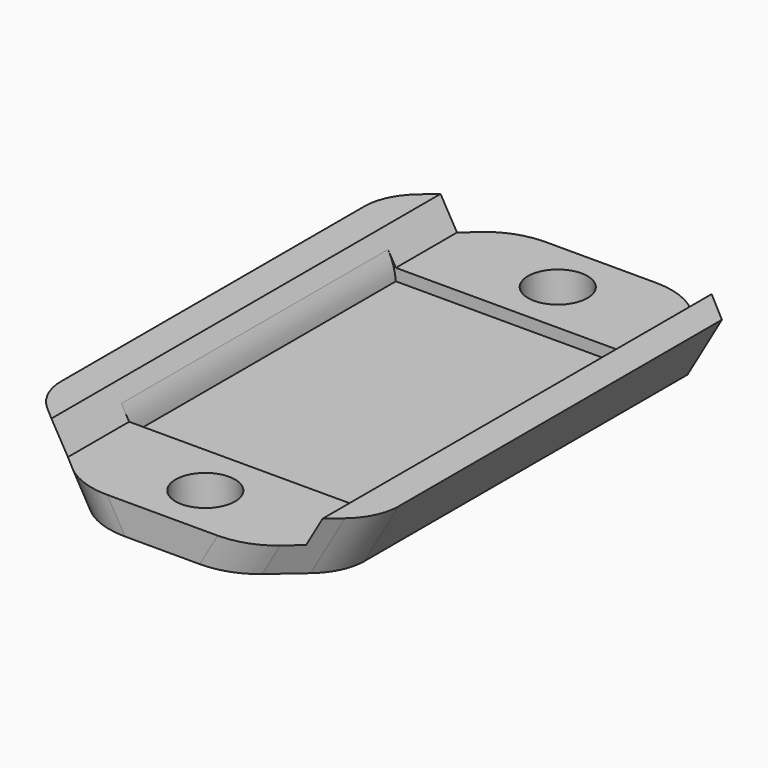
from build123d import *

# Parameters (mm, degrees)
F1_DEPTH    = 23
F2_W        = 20
F2_H        = 28
F3_DEPTH    = 1
F4_D        = 5
F5_SIZE     = 5
F6_T1_DEPTH = 28
F6_T3_DEPTH = 13.3575604591
F6_T5_DEPTH = 13.3575604591
F6_T7_DEPTH = 16.1288417512
F6_T9_DEPTH = 16.1288417512


# Not quite as in the source:
# - a fillet or chamfer that OpenCascade refuses, or shapes differently, is made with other operations: its cross-section is extruded or revolved along the edge and cut away or added


with BuildPart() as f1:
    # F0 (on Front) → F1 (new body, symmetric)
    with BuildSketch(Plane.XZ):
        Polygon((-11.2988893001, 0), (0, 0), (11.2988893001, 0), (14.1856406461, 5), (11.3856406461, 5), (10, 2.6), (0, 2.6), (-10, 2.6), (-11.3856406461, 5), (-14.1856406461, 5), align=None)
    extrude(amount=F1_DEPTH, both=True)

    # F2 (on face) → F3 (cut)
    with BuildSketch(Plane.XY.offset(2.6)):
        Rectangle(F2_W, F2_H)
    extrude(amount=-F3_DEPTH, mode=Mode.SUBTRACT)

    # F4 (through all)
    with Locations(Plane.XY.offset(2.6)):
        with Locations((0, -18.5), (0, 18.5)):
            Hole(F4_D / 2)

    # F5
    f5_edges = [f1.edges().sort_by_distance(p)[0] for p in [
        (-12.742265, -23, 2.5),
        (12.742265, -23, 2.5),
        (-12.742265, 23, 2.5),
        (12.742265, 23, 2.5),
    ]]
    chamfer(f5_edges, length=F5_SIZE)

    # F6: fillet of radius 5 on 9 edges, made by hand

    # F6_s2 → F6_t1 (cut)
    with BuildSketch(Plane.XZ.offset(-14)):
        with BuildLine():
            ThreePointArc((-10.656712034, 3.7374586088), (-10.2073363045, 2.7059113585), (-10, 1.6))
            Line((-10, 1.6), (-10, 2.6))
            Line((-10, 2.6), (-10.656712034, 3.7374586088))
        make_face()
        with BuildLine():
            ThreePointArc((10.656712034, 3.7374586088), (10.2073363045, 2.7059113585), (10, 1.6))
            Line((10, 1.6), (10, 2.6))
            Line((10, 2.6), (10.656712034, 3.7374586088))
        make_face()
    extrude(amount=F6_T1_DEPTH, mode=Mode.SUBTRACT)

    # F6_s4 → F6_t3 (cut)
    with BuildSketch(Plane(origin=(-5.4712921168, 0, 9.4765559293), x_dir=(0, 1, 0), z_dir=(0.5, 0, -0.8660254038))):
        with BuildLine():
            ThreePointArc((23, -2.7140573566), (22.6193976626, -4.6274745184), (21.5355339059, -6.2495912625))
            Line((21.5355339059, -6.2495912625), (23, -4.7851251684))
            Line((23, -4.7851251684), (23, -2.7140573566))
        make_face()
        with BuildLine():
            ThreePointArc((-21.5355339059, -6.2495912625), (-22.6193976626, -4.6274745184), (-23, -2.7140573566))
            Line((-23, -2.7140573566), (-23, -4.7851251684))
            Line((-23, -4.7851251684), (-21.5355339059, -6.2495912625))
        make_face()
    extrude(amount=F6_T3_DEPTH, mode=Mode.SUBTRACT)

    # F6_s6 → F6_t5 (cut)
    with BuildSketch(Plane(origin=(-1.2074881128, 0, -2.0914307609), x_dir=(0, 1, 0), z_dir=(0.5, 0, 0.8660254038))):
        with BuildLine():
            ThreePointArc((23, -2.7140573566), (22.6193976626, -4.6274745184), (21.5355339059, -6.2495912625))
            Line((21.5355339059, -6.2495912625), (23, -4.7851251684))
            Line((23, -4.7851251684), (23, -2.7140573566))
        make_face()
        with BuildLine():
            ThreePointArc((-21.5355339059, -6.2495912625), (-22.6193976626, -4.6274745184), (-23, -2.7140573566))
            Line((-23, -2.7140573566), (-23, -4.7851251684))
            Line((-23, -4.7851251684), (-21.5355339059, -6.2495912625))
        make_face()
    extrude(amount=F6_T5_DEPTH, mode=Mode.SUBTRACT)

    # F6_s8 → F6_t7 (cut)
    with BuildSketch(Plane(origin=(-8.3003084358, 0, 14.3765559293), x_dir=(0, 1, 0), z_dir=(0.5, 0, -0.8660254038))):
        with BuildLine():
            ThreePointArc((19.4644660941, -8.3206590744), (17.84234935, -9.404522831), (15.9289321881, -9.7851251684))
            Line((15.9289321881, -9.7851251684), (18, -9.7851251684))
            Line((18, -9.7851251684), (19.4644660941, -8.3206590744))
        make_face()
        with BuildLine():
            ThreePointArc((-15.9289321881, -9.7851251684), (-17.84234935, -9.404522831), (-19.4644660941, -8.3206590744))
            Line((-19.4644660941, -8.3206590744), (-18, -9.7851251684))
            Line((-18, -9.7851251684), (-15.9289321881, -9.7851251684))
        make_face()
    extrude(amount=F6_T7_DEPTH, mode=Mode.SUBTRACT)

    # F6_s10 → F6_t9 (cut)
    with BuildSketch(Plane(origin=(0.2358875602, 0, 0.4085692391), x_dir=(0, 1, 0), z_dir=(0.5, 0, 0.8660254038))):
        with BuildLine():
            ThreePointArc((-15.9289321881, -9.7851251684), (-17.84234935, -9.404522831), (-19.4644660941, -8.3206590744))
            Line((-19.4644660941, -8.3206590744), (-18, -9.7851251684))
            Line((-18, -9.7851251684), (-15.9289321881, -9.7851251684))
        make_face()
    extrude(amount=F6_T9_DEPTH, mode=Mode.SUBTRACT)


solid = f1.part
